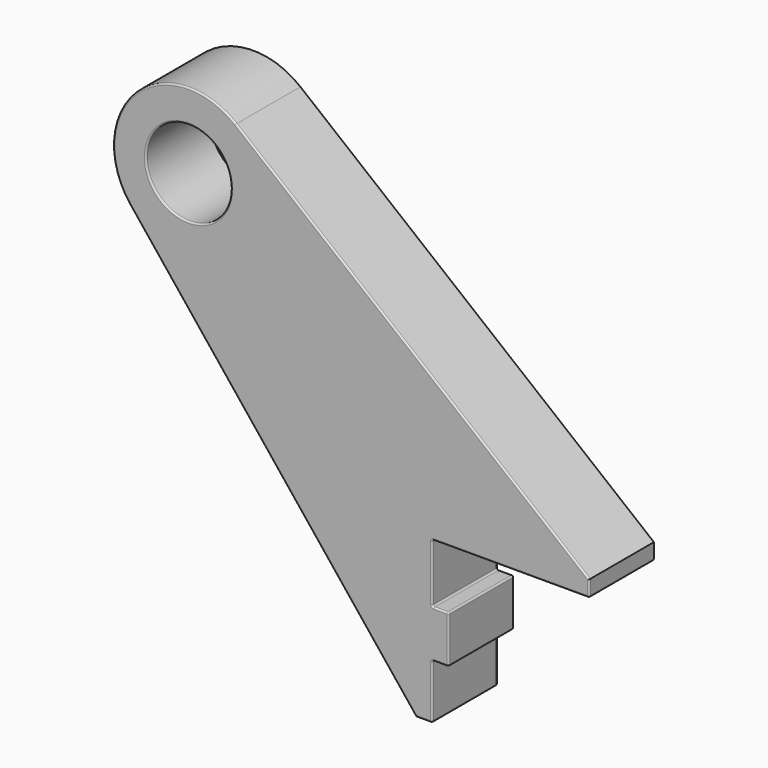
from build123d import *

# Parameters (mm, degrees)
F0_R     = 5.2
F1_DEPTH = 10
F2_R     = 0.2


with BuildPart() as f1:
    # F0 (on Front) → F1 (new body)
    with BuildSketch(Plane.XZ):
        Polygon((2.9, 10.1), (9.1, 10.1), (9.1, 12.1), (-12.1, 12.1), (-12.1, -9.6), (-10.1, -9.6), (-10.1, -2.9), (-8.1, -2.9), (-8.1, 2.9), (-10.1, 2.9), (-10.1, 10.1), (-2.9, 10.1), align=None)
        with BuildLine():
            Line((-12.1, 12.1), (9.1, 12.1))
            Line((9.1, 12.1), (-34.1143752893, 47.0530795261))
            ThreePointArc((-34.1143752893, 47.0530795261), (-31.5973574285, 43.863095549), (-30.7, 39.9))
            ThreePointArc((-30.7, 39.9), (-36.8558404571, 31.2182321686), (-47.0854549299, 34.1546333929))
            Line((-47.0854549299, 34.1546333929), (-12.1, -9.6))
            Line((-12.1, -9.6), (-12.1, 12.1))
        make_face()
        with BuildLine():
            ThreePointArc((-30.7, 39.9), (-31.5973574285, 43.863095549), (-34.1143752893, 47.0530795261))
            ThreePointArc((-34.1143752893, 47.0530795261), (-46.3870917462, 46.4236217454), (-47.0854549299, 34.1546333929))
            ThreePointArc((-47.0854549299, 34.1546333929), (-36.8558404571, 31.2182321686), (-30.7, 39.9))
        make_face()
        with Locations((-39.9, 39.9)):
            Circle(F0_R, mode=Mode.SUBTRACT)
    extrude(amount=F1_DEPTH)

    # F2
    f2_edges = [f1.edges().sort_by_distance(p)[0] for p in [
        (-8.1, -5, -2.9),
        (-8.1, -5, 2.9),
        (-8.1, 0, 0),
        (-8.1, -10, 0),
        (-10.1, -5, 2.9),
        (-10.1, -5, 10.1),
        (-10.1, 0, 6.5),
        (-10.1, -10, 6.5),
        (-10.1, -5, -9.6),
        (-10.1, -5, -2.9),
        (-10.1, 0, -6.25),
        (-10.1, -10, -6.25),
        (9.1, -5, 10.1),
        (-0.5, 0, 10.1),
        (-0.5, -10, 10.1),
        (9.1, 0, 11.1),
        (-12.507188, 0, 29.57654),
        (-46.387092, 0, 46.423622),
        (-29.592727, 0, 12.277317),
        (-11.1, 0, -9.6),
        (-9.1, 0, -2.9),
        (-9.1, 0, 2.9),
        (-45.1, 0, 39.9),
        (9.1, -10, 11.1),
        (-12.507188, -10, 29.57654),
        (-46.387092, -10, 46.423622),
        (-29.592727, -10, 12.277317),
        (-11.1, -10, -9.6),
        (-9.1, -10, -2.9),
        (-9.1, -10, 2.9),
        (-45.1, -10, 39.9),
    ]]
    fillet(f2_edges, radius=F2_R)


solid = f1.part
